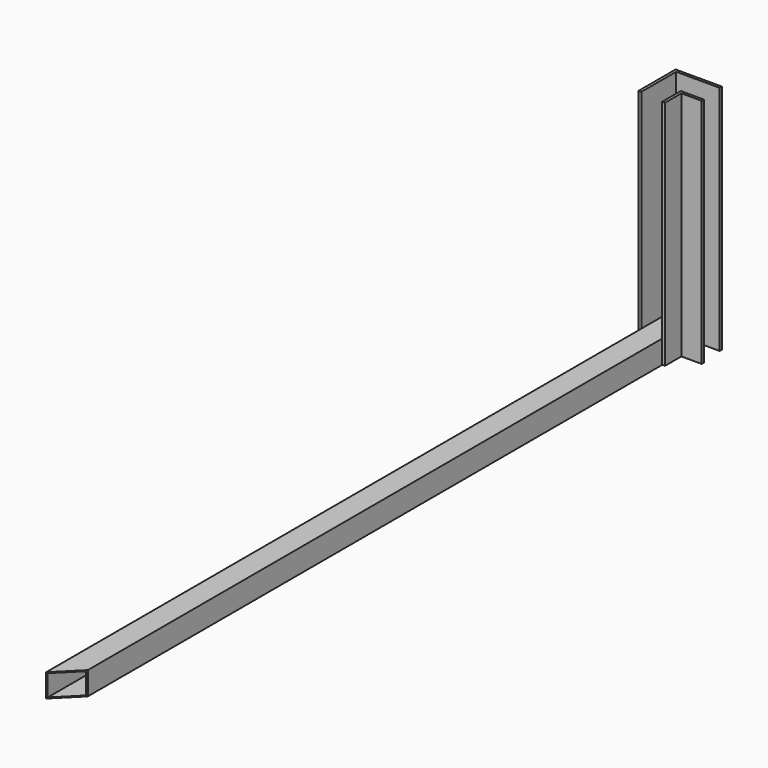
from build123d import *

# Parameters (mm, degrees)
F5_DEPTH = 50
F4_W     = 50
F4_H     = 50
F4_W_2   = 46
F4_H_2   = 46
F1_DEPTH = 850
F3_W     = 6
F3_H     = 6
F7_DEPTH = 500


# Not quite as in the source:
# - a feature names something its author has since deleted; it is built from what else it names


with BuildPart() as f5:
    # F0 (on Top) → F5 (new body)
    with BuildSketch(Plane.XY):
        Polygon((51, 0), (0, 0), (25.5, -25.5), align=None)
        Polygon((51, -51), (51, 0), (25.5, -25.5), align=None)
    extrude(amount=F5_DEPTH)


with BuildPart() as f1:
    # F4 (on Front) → F1 (new body)
    with BuildSketch(Plane.XZ):
        with Locations((25, 25)):
            Rectangle(F4_W, F4_H)
        with Locations((25, 25)):
            Rectangle(F4_W_2, F4_H_2, mode=Mode.SUBTRACT)
    extrude(amount=F1_DEPTH)

    # F2: cut F5
    add(f5.part, mode=Mode.SUBTRACT)

    # F6: F1 across face


with BuildPart() as f1_1:
    add(f1.part)
    add(f1.part.mirror(Plane(origin=(25, -850, 25), x_dir=(1, 0, 0), z_dir=(0, -1, 0))))


with BuildPart() as f7:
    # F3 (on Top) → F7 (new body)
    with BuildSketch(Plane.XY):
        Polygon((94, -56), (94, -50), (50, -50), (50, -94), (56, -94), (56, -56), align=None)
        with Locations((53, -97)):
            Rectangle(F3_W, F3_H)
        with Locations((97, -53)):
            Rectangle(F3_W, F3_H)
    extrude(amount=F7_DEPTH)


with BuildPart() as f7b:
    # F3 (on Top) → F7, piece 2 (new body)
    with BuildSketch(Plane.XY):
        Polygon((0, -94), (0, 0), (94, 0), (94, 6), (-6, 6), (-6, -94), align=None)
    extrude(amount=F7_DEPTH)


solid = Compound([f1_1.part, f7.part, f7b.part])
